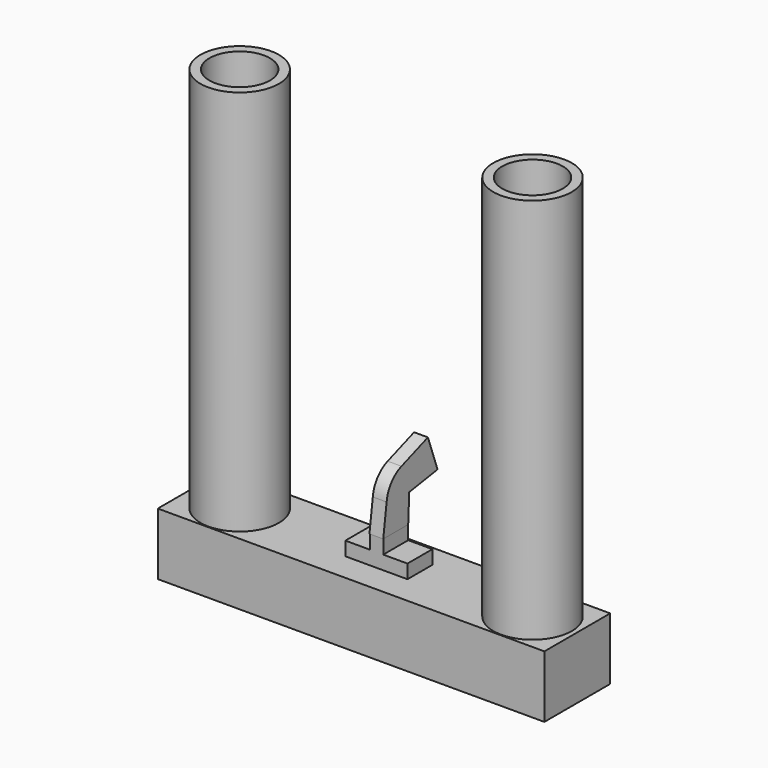
from build123d import *

# Parameters (mm, degrees)
F0_R     = 5.6894885444
F0_R_2   = 4.3843175031
F1_DEPTH = 65
F0_W     = 56.0123268515
F0_H     = 11.923417449
F2_DEPTH = 9
F3_W     = 9.0000643395
F3_H     = 4.5161172748
F4_DEPTH = 2
F5_W     = 1.888447674
F5_H     = 4.5161172748
F6_DEPTH = 2
F8_DEPTH = 2


with BuildPart() as f1:
    # F0 (on Top) → F1 (new body)
    with BuildSketch(Plane.XY):
        with Locations((-21.2125875842, 38.5669283569)):
            Circle(F0_R)
        with Locations((-21.2125875842, 38.5669283569)):
            Circle(F0_R_2, mode=Mode.SUBTRACT)
    extrude(amount=F1_DEPTH)



with BuildPart() as f1b:
    # F0 (on Top) → F1, piece 2 (new body)
    with BuildSketch(Plane.XY):
        with Locations((21.215147819, 38.5669283569)):
            Circle(F0_R)
        with Locations((21.215147819, 38.5669283569)):
            Circle(F0_R_2, mode=Mode.SUBTRACT)
    extrude(amount=F1_DEPTH)


with BuildPart() as f1_1:
    add(f1.part)

    add(f1b.part)  # F2 merges F1b
    # F0 (on Top) → F2 (join)
    with BuildSketch(Plane.XY):
        with Locations((-0.4159319069, 38.7055762112)):
            Rectangle(F0_W, F0_H)
        with Locations((-21.2125875842, 38.5669283569)):
            Circle(F0_R, mode=Mode.SUBTRACT)
        with Locations((21.215147819, 38.5669283569)):
            Circle(F0_R, mode=Mode.SUBTRACT)
    extrude(amount=F2_DEPTH)

    # F3 (on face) → F4 (join)
    with BuildSketch(Plane.XY.offset(9)):
        with Locations((-0.0426771585, 39.1226857901)):
            Rectangle(F3_W, F3_H)
    extrude(amount=F4_DEPTH)

    # F5 (on face) → F6 (join)
    with BuildSketch(Plane.XY.offset(11)):
        with Locations((0.0049760565, 39.1226857901)):
            Rectangle(F5_W, F5_H)
    extrude(amount=F6_DEPTH)


with BuildPart() as f8:
    # F7 (on face) → F8 (new body)
    with BuildSketch(Plane.YZ.offset(0.9491998935)):
        with BuildLine():
            Line((37.4740036153, 17.461272415), (36.8646271527, 13))
            Line((36.8646271527, 13), (41.3807444274, 13))
            Line((41.3807444274, 13), (41.5678136051, 17.0637406409))
            Line((41.5678136051, 17.0637406409), (46.4460814167, 17.8263583901))
            Line((46.4460814167, 17.8263583901), (46.6797463596, 17.9114900529))
            Line((46.6797463596, 17.9114900529), (44.94539564, 22.6718453473))
            Line((44.94539564, 22.6718453473), (40.1598270518, 20.9283086128))
            ThreePointArc((40.1598270518, 20.9283086128), (38.3162714633, 19.5826263954), (37.4740036153, 17.461272415))
        make_face()
    extrude(amount=-F8_DEPTH)


solid = Compound([f1_1.part, f8.part])
